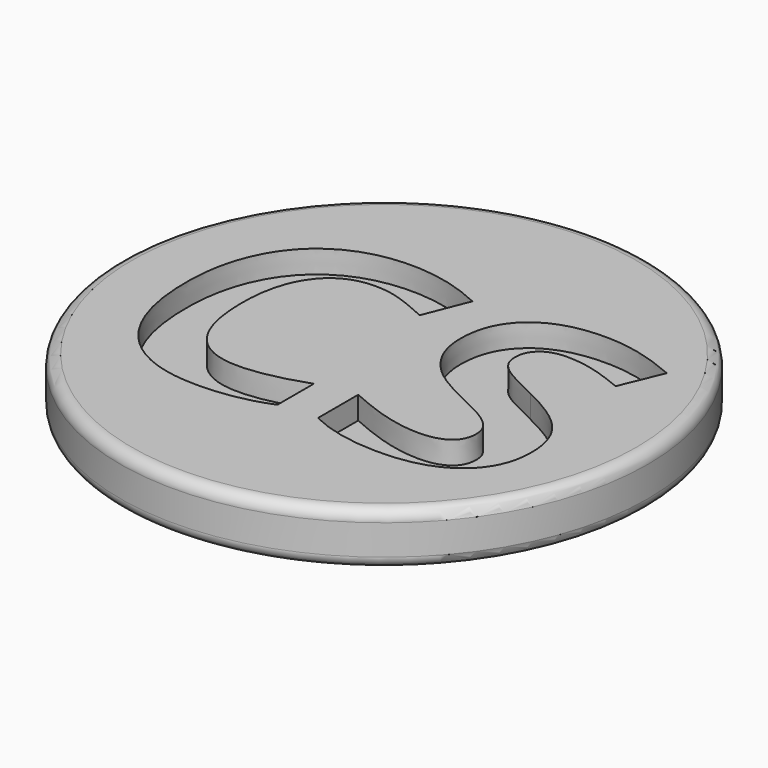
from build123d import *

# Parameters (mm, degrees)
F0_R         = 11.605
F1_DEPTH     = 1.165
F2_R         = 0.5
F3_TEXT_SIZE = 15.7447746337
F4_DEPTH     = 1


# Not quite as in the source:
# - Text() gives the source's letters only with a copy of the font that has no kerning and outlines rounded to 1/6400 em; it was checked with that copy


with BuildPart() as f1:
    # F0 (on Top) → F1 (new body, symmetric)
    with BuildSketch(Plane.XY):
        Circle(F0_R)
    extrude(amount=F1_DEPTH, both=True)

    # F2
    f2_edges = [f1.edges().sort_by_distance(p)[0] for p in [
        (-11.605, 0, -1.165),
        (-11.605, 0, 1.165),
    ]]
    fillet(f2_edges, radius=F2_R)

    # F3 (on face) → F4 (cut)
    with BuildSketch(Plane.XY.offset(1.165)):
        with Locations((-9.5514199243, -5.6649273985)):
            Text('CS', F3_TEXT_SIZE, font='Open Sans', font_style=FontStyle.BOLD, text_align=(TextAlign.LEFT, TextAlign.BOTTOM))
    extrude(amount=-F4_DEPTH, mode=Mode.SUBTRACT)


solid = f1.part
